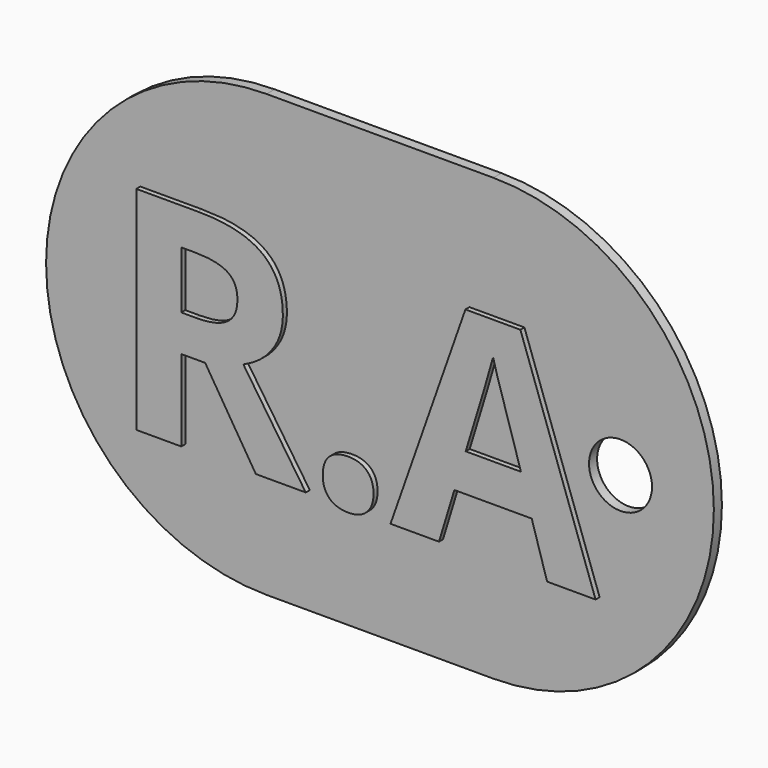
from build123d import *

# Parameters (mm, degrees)
F0_R         = 3.175
F1_DEPTH     = 1.016
F2_TEXT_SIZE = 29.9571961578
F3_DEPTH     = 1.524


# Not quite as in the source:
# - Text() gives the source's letters only with a copy of the font that has no kerning and outlines rounded to 1/6400 em; it was checked with that copy


with BuildPart() as f1:
    # F0 (on Front) → F1 (new body)
    with BuildSketch(Plane.XZ):
        with BuildLine():
            Line((-29.9253943107, 22.225), (-52.7853943107, 22.225))
            ThreePointArc((-52.7853943107, 22.225), (-75.0103943107, 0), (-52.7853943107, -22.225))
            Line((-52.7853943107, -22.225), (-29.9253943107, -22.225))
            ThreePointArc((-29.9253943107, -22.225), (-7.7003943107, 0), (-29.9253943107, 22.225))
        make_face()
        with Locations((-17.10877195, 0)):
            Circle(F0_R, mode=Mode.SUBTRACT)
    extrude(amount=F1_DEPTH)

    # F2 (on Front) → F3 (join)
    with BuildSketch(Plane.XZ):
        with Locations((-68.2052522898, -11.5132806823)):
            Text('R.A', F2_TEXT_SIZE, font='Open Sans', font_style=FontStyle.BOLD, text_align=(TextAlign.LEFT, TextAlign.BOTTOM))
    extrude(amount=F3_DEPTH)


solid = f1.part
